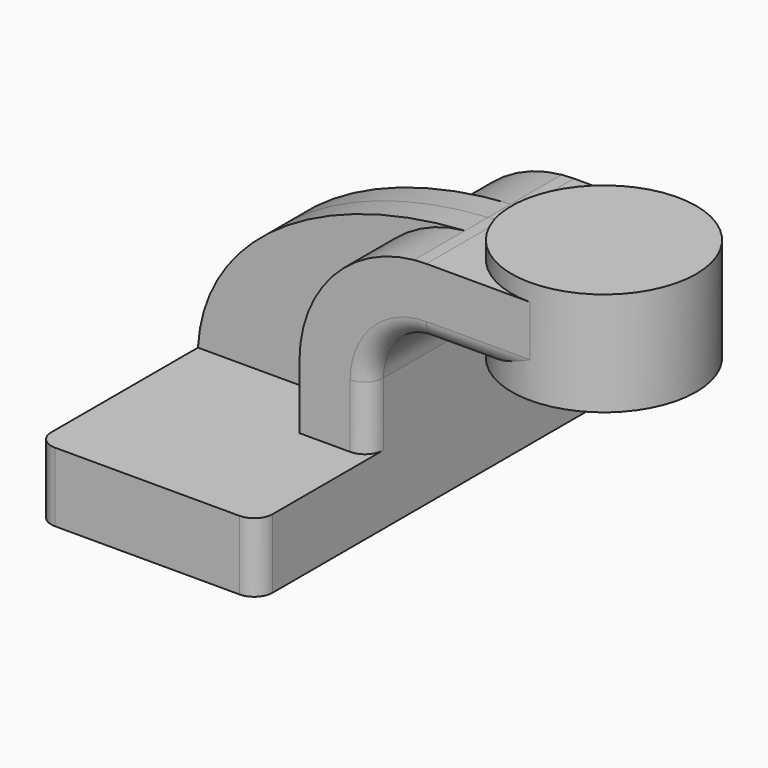
from build123d import *

# Parameters (mm, degrees)
F1_DEPTH     = 63.5
F0_W         = 25.4
F0_H         = 19.05
F2_DEPTH     = 25.4
F3_DEPTH     = 7.9375
F5_R         = 5.08
F6_T1_DEPTH  = 17.4752
F6_T6_DEPTH  = 50.165
F6_S7_R      = 25.4
F6_T8_DEPTH  = 27
F6_T10_ANGLE = 90
F7_T1_DEPTH  = 17.4752
F7_T6_DEPTH  = 50.165
F7_S7_R      = 25.4
F7_T8_DEPTH  = 27
F7_T10_ANGLE = 90


# Not quite as in the source:
# - a fillet or chamfer that OpenCascade refuses, or shapes differently, is made with other operations: its cross-section is extruded or revolved along the edge and cut away or added


with BuildPart() as f1:
    # F0 (on Front) → F1 (new body, symmetric)
    with BuildSketch(Plane.XZ):
        Polygon((11.43, 9.525), (-30.48, 9.525), (-30.48, -9.525), (30.48, -9.525), (30.48, 9.525), align=None)
    extrude(amount=F1_DEPTH, both=True)

    # F0 (on Front) → F2 (join, symmetric)
    with BuildSketch(Plane.XZ):
        with BuildLine():
            Line((11.43, 27.0002), (11.43, 9.525))
            Line((11.43, 9.525), (30.48, 9.525))
            Line((30.48, 9.525), (30.48, 27.0002))
            ThreePointArc((30.48, 27.0002), (35.1296798487, 38.2255201513), (46.355, 42.8752))
            Line((46.355, 42.8752), (49.53, 42.8752))
            Line((49.53, 42.8752), (49.53, 61.9252))
            Line((49.53, 61.9252), (46.355, 61.9252))
            add(Edge.make_bspline(
                [(43.0102942151, 61.7646727878), (44.1205521815, 61.8325692622), (45.2356507943, 61.8861371605), (46.355, 61.9252)],
                knots=[90.4192998356, 90.4192998356, 90.4192998356, 90.4192998356, 93.0021407551, 93.0021407551, 93.0021407551, 93.0021407551], degree=3))
            ThreePointArc((43.0102942151, 61.7646727878), (20.5037962124, 50.4836172925), (11.43, 27.0002))
        make_face()
        with Locations((62.23, 52.4002)):
            Rectangle(F0_W, F0_H)
    extrude(amount=F2_DEPTH, both=True)

    # F0 (on Front) → F3 (join, symmetric)
    with BuildSketch(Plane.XZ):
        with BuildLine():
            add(Edge.make_bspline(
                [(-30.48, 9.525), (-28.7924455478, 39.4506532923), (4.142725098, 59.3877739136), (43.0102942151, 61.7646727878)],
                knots=[0, 0, 0, 0, 90.4192998356, 90.4192998356, 90.4192998356, 90.4192998356], degree=3))
            Line((-30.48, 9.525), (11.43, 9.525))
            Line((11.43, 9.525), (11.43, 27.0002))
            ThreePointArc((11.43, 27.0002), (20.5037962124, 50.4836172925), (43.0102942151, 61.7646727878))
        make_face()
    extrude(amount=F3_DEPTH, both=True)

    # F0 (on Front) → F4 (revolve)
    with BuildSketch(Plane.XZ):
        Polygon((74.93, 66.675), (74.93, 61.9252), (74.93, 42.8752), (74.93, 38.1), (100.33, 38.1), (100.33, 66.675), align=None)
    revolve(axis=Axis((74.93, 0, 52.3875), (0, 0, 1)))

    # F5
    f5_edges = [f1.edges().sort_by_distance(p)[0] for p in [
        (30.48, -63.5, 0),
        (-30.48, -63.5, 0),
        (30.48, 63.5, 0),
        (-30.48, 63.5, 0),
    ]]
    fillet(f5_edges, radius=F5_R)

    # F6: fillet of radius 5.08 on 1 edges, made by hand

    # F6_s2 → F6_t1 (cut)
    with BuildSketch(Plane.XY.offset(9.525)):
        with BuildLine():
            ThreePointArc((30.48, -20.32), (28.9921024484, -23.9121024484), (25.4, -25.4))
            Line((25.4, -25.4), (30.48, -25.4))
            Line((30.48, -25.4), (30.48, -20.32))
        make_face()
    extrude(amount=F6_T1_DEPTH, mode=Mode.SUBTRACT)


with BuildPart() as f6_tool4:
    # F6_s5 → F6_t6 (new body)
    with BuildSketch(Plane.YZ.offset(46.355)):
        with BuildLine():
            ThreePointArc((-25.4, 47.9552), (-23.9121024484, 44.3630975516), (-20.32, 42.8752))
            Line((-20.32, 42.8752), (-25.4, 42.8752))
            Line((-25.4, 42.8752), (-25.4, 47.9552))
        make_face()
    extrude(amount=F6_T6_DEPTH)

    # F6_s7 → F6_t8 (cut, symmetric)
    with BuildSketch(Plane.XY.offset(45.4)):
        with Locations((74.93, 0)):
            Circle(F6_S7_R)
    extrude(amount=F6_T8_DEPTH, both=True, mode=Mode.SUBTRACT)


with BuildPart() as f1_1:
    add(f1.part)

    # F6_t3: cut F6_tool4
    add(f6_tool4.part, mode=Mode.SUBTRACT)

    # F6_s9 → F6_t10 (revolve, cut)
    with BuildSketch(Plane.XY.offset(27.0002)):
        with BuildLine():
            ThreePointArc((30.48, -20.32), (28.9921024484, -23.9121024484), (25.4, -25.4))
            Line((25.4, -25.4), (30.48, -25.4))
            Line((30.48, -25.4), (30.48, -20.32))
        make_face()
    revolve(axis=Axis((46.355, -25.4, 27.0002), (0, 1, 0)), revolution_arc=F6_T10_ANGLE, mode=Mode.SUBTRACT)

    # F7: fillet of radius 5.08 on 3 edges, made by hand

    # F7_s2 → F7_t1 (cut)
    with BuildSketch(Plane.XY.offset(9.525)):
        with BuildLine():
            ThreePointArc((30.48, 20.32), (28.9921024484, 23.9121024484), (25.4, 25.4))
            Line((25.4, 25.4), (30.48, 25.4))
            Line((30.48, 25.4), (30.48, 20.32))
        make_face()
    extrude(amount=F7_T1_DEPTH, mode=Mode.SUBTRACT)


with BuildPart() as f7_tool4:
    # F7_s5 → F7_t6 (new body)
    with BuildSketch(Plane.YZ.offset(46.355)):
        with BuildLine():
            ThreePointArc((25.4, 47.9552), (23.9121024484, 44.3630975516), (20.32, 42.8752))
            Line((20.32, 42.8752), (25.4, 42.8752))
            Line((25.4, 42.8752), (25.4, 47.9552))
        make_face()
    extrude(amount=F7_T6_DEPTH)

    # F7_s7 → F7_t8 (cut, symmetric)
    with BuildSketch(Plane.XY.offset(45.4)):
        with Locations((74.93, 0)):
            Circle(F7_S7_R)
    extrude(amount=F7_T8_DEPTH, both=True, mode=Mode.SUBTRACT)


with BuildPart() as f1_2:
    add(f1_1.part)

    # F7_t3: cut F7_tool4
    add(f7_tool4.part, mode=Mode.SUBTRACT)

    # F7_s9 → F7_t10 (revolve, cut)
    with BuildSketch(Plane.XY.offset(27.0002)):
        with BuildLine():
            ThreePointArc((25.4, 25.4), (28.9921024484, 23.9121024484), (30.48, 20.32))
            Line((30.48, 20.32), (30.48, 25.4))
            Line((30.48, 25.4), (25.4, 25.4))
        make_face()
    revolve(axis=Axis((46.355, 25.4, 27.0002), (0, 1, 0)), revolution_arc=F7_T10_ANGLE, mode=Mode.SUBTRACT)


solid = f1_2.part
